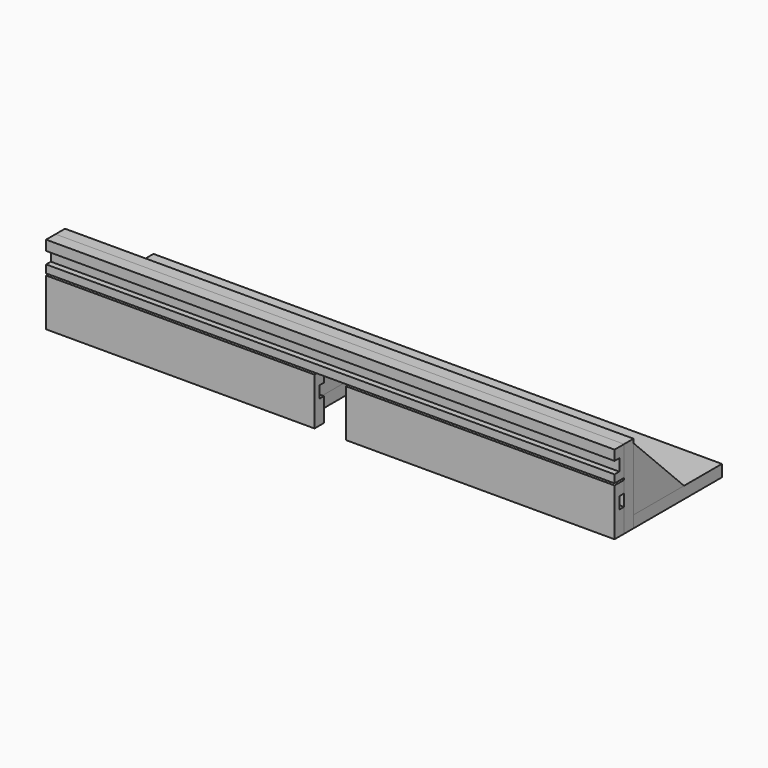
from build123d import *

# Parameters (mm, degrees)
F0_W      = 914.4
F0_H      = 177.8
F1_DEPTH  = 19.05
F2_W      = 914.4
F2_H      = 19.05
F3_DEPTH  = 127
F4_W      = 431.8
F4_H      = 76.2
F5_DEPTH  = 19.05
F6_W      = 914.4
F6_H      = 47.752
F7_DEPTH  = 19.05
F8_W      = 9.525
F8_H      = 19.05
F9_DEPTH  = 914.4
F10_W     = 19.05
F10_H     = 101.6
F11_DEPTH = 101.6
F13_DEPTH = 914.4
F14_W     = 101.6
F14_H     = 82.55
F14_H_2   = 19.05
F15_DEPTH = 73.152
F16_W     = 9.525
F16_H     = 19.05
F17_DEPTH = 914.4
F18_R     = 4.191
F19_DEPTH = 19.05
F21_DEPTH = 19.05


# Not quite as in the source:
# - a feature names something its author has since deleted; it is built from what else it names


with BuildPart() as f1:
    # F0 (on Top) → F1 (new body)
    with BuildSketch(Plane.XY):
        with Locations((0, -19.3418145372)):
            Rectangle(F0_W, F0_H)
    extrude(amount=F1_DEPTH)


with BuildPart() as f3:
    # F2 (on face) → F3 (new body)
    with BuildSketch(Plane(origin=(0, 0, 0), x_dir=(1, 0, 0), z_dir=(0, 0, -1))):
        with Locations((0, 117.7668145372)):
            Rectangle(F2_W, F2_H)
    extrude(amount=-F3_DEPTH)


with BuildPart() as f5:
    # F4 (on face) → F5 (new body)
    with BuildSketch(Plane.XZ.offset(127.2918145372)):
        with Locations((-241.3, 38.1)):
            Rectangle(F4_W, F4_H)
    extrude(amount=F5_DEPTH)


with BuildPart() as f5b:
    # F4 (on face) → F5, piece 2 (new body)
    with BuildSketch(Plane.XZ.offset(127.2918145372)):
        with Locations((241.3, 38.1)):
            Rectangle(F4_W, F4_H)
    extrude(amount=F5_DEPTH)


with BuildPart() as f7:
    # F6 (on face) → F7 (new body)
    with BuildSketch(Plane.XZ.offset(127.2918145372)):
        with Locations((0, 103.124)):
            Rectangle(F6_W, F6_H)
    extrude(amount=F7_DEPTH)

    # F8 (on face) → F9 (cut, through all)
    with BuildSketch(Plane.YZ.offset(457.2)):
        with Locations((-141.5793145372, 101.473)):
            Rectangle(F8_W, F8_H)
    extrude(amount=-F9_DEPTH, mode=Mode.SUBTRACT)


with BuildPart() as f11:
    # F10 (on face) → F11 (new body)
    with BuildSketch(Plane.XY.offset(19.05)):
        with Locations((-447.675, -57.4418145372)):
            Rectangle(F10_W, F10_H)
    extrude(amount=F11_DEPTH)


with BuildPart() as f11b:
    # F10 (on face) → F11, piece 2 (new body)
    with BuildSketch(Plane.XY.offset(19.05)):
        with Locations((-257.175, -57.4418145372)):
            Rectangle(F10_W, F10_H)
    extrude(amount=F11_DEPTH)


with BuildPart() as f11c:
    # F10 (on face) → F11, piece 3 (new body)
    with BuildSketch(Plane.XY.offset(19.05)):
        with Locations((-60.325, -57.4418145372)):
            Rectangle(F10_W, F10_H)
    extrude(amount=F11_DEPTH)


with BuildPart() as f11d:
    # F10 (on face) → F11, piece 4 (new body)
    with BuildSketch(Plane.XY.offset(19.05)):
        with Locations((60.325, -57.4418145372)):
            Rectangle(F10_W, F10_H)
    extrude(amount=F11_DEPTH)


with BuildPart() as f11e:
    # F10 (on face) → F11, piece 5 (new body)
    with BuildSketch(Plane.XY.offset(19.05)):
        with Locations((257.175, -57.4418145372)):
            Rectangle(F10_W, F10_H)
    extrude(amount=F11_DEPTH)


with BuildPart() as f11f:
    # F10 (on face) → F11, piece 6 (new body)
    with BuildSketch(Plane.XY.offset(19.05)):
        with Locations((447.675, -57.4418145372)):
            Rectangle(F10_W, F10_H)
    extrude(amount=F11_DEPTH)


with BuildPart() as f13_tool:
    # F12 (on face) → F13 (new body, through all)
    with BuildSketch(Plane(origin=(-457.2, 0, 0), x_dir=(0, -1, 0), z_dir=(-1, 0, 0))):
        Polygon((6.6418145372, 120.65), (6.6418145372, 19.05), (108.2418145372, 120.65), align=None)
    extrude(amount=-F13_DEPTH)


with BuildPart() as f11_1:
    add(f11.part)

    # F13: cut by f13_tool
    add(f13_tool.part, mode=Mode.SUBTRACT)


with BuildPart() as f11b_1:
    add(f11b.part)

    # F13: cut by f13_tool
    add(f13_tool.part, mode=Mode.SUBTRACT)


with BuildPart() as f11c_1:
    add(f11c.part)

    # F13: cut by f13_tool
    add(f13_tool.part, mode=Mode.SUBTRACT)


with BuildPart() as f11d_1:
    add(f11d.part)

    # F13: cut by f13_tool
    add(f13_tool.part, mode=Mode.SUBTRACT)


with BuildPart() as f11e_1:
    add(f11e.part)

    # F13: cut by f13_tool
    add(f13_tool.part, mode=Mode.SUBTRACT)


with BuildPart() as f11f_1:
    add(f11f.part)

    # F13: cut by f13_tool
    add(f13_tool.part, mode=Mode.SUBTRACT)


with BuildPart() as f15_tool:
    # F14 (on face) → F15 (new body)
    with BuildSketch(Plane(origin=(0, 0, 0), x_dir=(1, 0, 0), z_dir=(0, 0, -1))):
        with Locations((0, 66.9668145372)):
            Rectangle(F14_W, F14_H)
        with Locations((0, 117.7668145372)):
            Rectangle(F14_W, F14_H_2)
    extrude(amount=-F15_DEPTH)


with BuildPart() as f1_1:
    add(f1.part)

    # F15: cut by f15_tool
    add(f15_tool.part, mode=Mode.SUBTRACT)

    # F20 (on face) → F21 (cut, through all)
    with BuildSketch(Plane.XY.offset(19.05)):
        Polygon((-254, 35.6491854628), (-273.05, 35.6491854628), (-292.1, 35.6491854628), (-292.1, 27.2671854628), (-254, 27.2671854628), align=None)
        Polygon((292.1, 35.6491854628), (273.05, 35.6491854628), (254, 35.6491854628), (254, 27.2671854628), (292.1, 27.2671854628), align=None)
    extrude(amount=-F21_DEPTH, mode=Mode.SUBTRACT)


with BuildPart() as f3_1:
    add(f3.part)

    # F15: cut by f15_tool
    add(f15_tool.part, mode=Mode.SUBTRACT)

    # F18 (on face) → F19 (cut)
    with BuildSketch(Plane(origin=(0, -108.2418145372, 0), x_dir=(-1, 0, 0), z_dir=(0, 1, 0))):
        with Locations((-355.6, 47.625)):
            Circle(F18_R)
        with Locations((158.75, 47.625)):
            Circle(F18_R)
        with Locations((355.6, 47.625)):
            Circle(F18_R)
        with Locations((-158.75, 47.625)):
            Circle(F18_R)
    extrude(amount=-F19_DEPTH, mode=Mode.SUBTRACT)


with BuildPart() as f17_tool:
    # F16 (on face) → F17 (new body, through all)
    with BuildSketch(Plane.YZ.offset(457.2)):
        with Locations((-132.0543145372, 47.625)):
            Rectangle(F16_W, F16_H)
    extrude(amount=-F17_DEPTH)


with BuildPart() as f5_1:
    add(f5.part)

    # F17: cut by f17_tool
    add(f17_tool.part, mode=Mode.SUBTRACT)


with BuildPart() as f5b_1:
    add(f5b.part)

    # F17: cut by f17_tool
    add(f17_tool.part, mode=Mode.SUBTRACT)


solid = Compound([f7.part, f11_1.part, f11b_1.part, f11c_1.part, f11d_1.part, f11e_1.part, f11f_1.part, f1_1.part, f3_1.part, f5_1.part, f5b_1.part])
